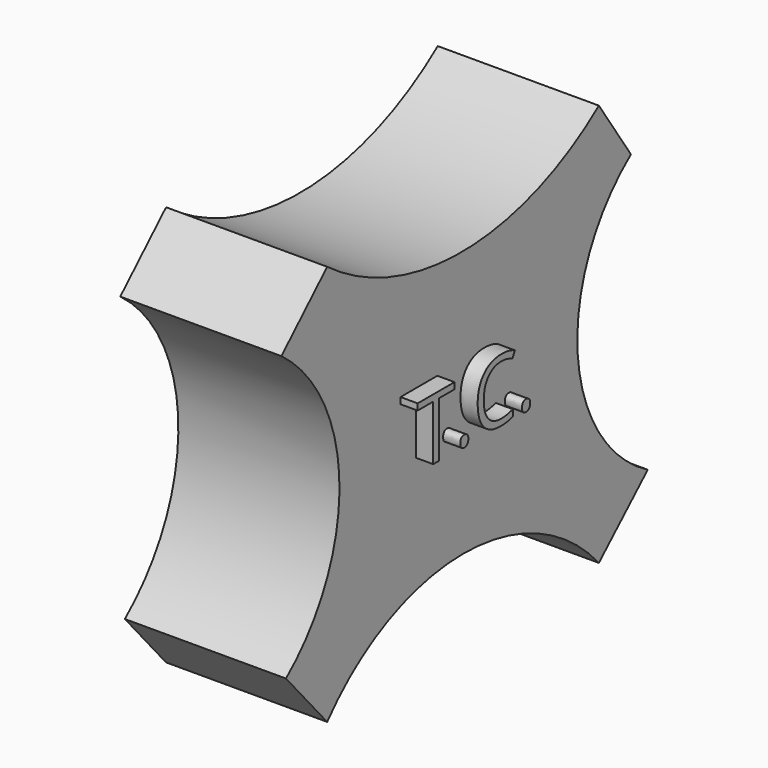
from build123d import *

# Parameters (mm, degrees)
F0_R         = 31.675863552
F0_R_2       = 20.376130664
F1_DEPTH     = 25.4
F0_R_3       = 31.7015587756
F0_R_4       = 20.4227004941
F0_R_5       = 31.6915672548
F0_R_6       = 20.4404132929
F0_R_7       = 31.6458572946
F0_R_8       = 20.0719257162
F3_DEPTH     = 25.4
F4_T         = -2.5
F4_2_T       = -2.5
F4_3_T       = -2.5
F4_4_T       = -2.5
F9_TEXT_SIZE = 13.5690788738
F10_DEPTH    = 28.1


# Not quite as in the source:
# - Text() gives the source's letters only with a copy of the font that has no kerning and outlines rounded to 1/6400 em; it was checked with that copy


with BuildPart() as f1:
    # F0 (on Front) → F1 (new body)
    with BuildSketch(Plane.XZ):
        with Locations((-40.9073680639, 37.5986844301)):
            Circle(F0_R)
        with Locations((-40.9073680639, 37.5986844301)):
            Circle(F0_R_2, mode=Mode.SUBTRACT)
    extrude(amount=F1_DEPTH)

    # F4
    f4_openings = [f1.faces().sort_by_distance(p)[0] for p in [
        (-71.687303, -25.4, 37.598684),
    ]]
    offset(amount=F4_T, openings=f4_openings)


with BuildPart() as f1b:
    # F0 (on Front) → F1, piece 2 (new body)
    with BuildSketch(Plane.XZ):
        with Locations((37.8994755447, 37.5986844301)):
            Circle(F0_R_3)
        with Locations((37.8994755447, 37.5986844301)):
            Circle(F0_R_4, mode=Mode.SUBTRACT)
    extrude(amount=F1_DEPTH)

    # F4#2
    f4_2_openings = [f1b.faces().sort_by_distance(p)[0] for p in [
        (7.094572, -25.4, 37.598684),
    ]]
    offset(amount=F4_2_T, openings=f4_2_openings)


with BuildPart() as f1c:
    # F0 (on Front) → F1, piece 3 (new body)
    with BuildSketch(Plane.XZ):
        with Locations((37.8994755447, -36.696318537)):
            Circle(F0_R_5)
        with Locations((37.8994755447, -36.696318537)):
            Circle(F0_R_6, mode=Mode.SUBTRACT)
    extrude(amount=F1_DEPTH)

    # F4#4
    f4_4_openings = [f1c.faces().sort_by_distance(p)[0] for p in [
        (7.104281, -25.4, -36.696319),
    ]]
    offset(amount=F4_4_T, openings=f4_4_openings)


with BuildPart() as f1d:
    # F0 (on Front) → F1, piece 4 (new body)
    with BuildSketch(Plane.XZ):
        with Locations((-40.9073680639, -36.696318537)):
            Circle(F0_R_7)
        with Locations((-40.9073680639, -36.696318537)):
            Circle(F0_R_8, mode=Mode.SUBTRACT)
    extrude(amount=F1_DEPTH)

    # F4#3
    f4_3_openings = [f1d.faces().sort_by_distance(p)[0] for p in [
        (-71.658145, -25.4, -36.696319),
    ]]
    offset(amount=F4_3_T, openings=f4_3_openings)


with BuildPart() as f3:
    # F2 (on Right) → F3 (new body)
    with BuildSketch(Plane.YZ):
        with BuildLine():
            ThreePointArc((64.6697282791, 31.2821045518), (38.0009545406, 21.9491823139), (11.1292116344, 30.6805260479))
            Line((11.1292116344, 30.6805260479), (2.1055291872, 21.9491823139))
            ThreePointArc((2.1055291872, 21.9491823139), (13.545850262, -0.3859795657), (3.0078974087, -23.1607891619))
            Line((3.0078974087, -23.1607891619), (11.1292116344, -32.4852652848))
            ThreePointArc((11.1292116344, -32.4852652848), (37.8303737781, -20.0358192392), (64.6697282791, -32.1844741702))
            Line((64.6697282791, -32.1844741702), (74.2950066924, -23.1607891619))
            ThreePointArc((74.2950066924, -23.1607891619), (60.495703437, -1.4966005988), (70.9863230586, 21.9491823139))
            Line((70.9863230586, 21.9491823139), (64.6697282791, 31.2821045518))
        make_face()
    extrude(amount=F3_DEPTH)

    # F9 (on Right) → F10 (join)
    with BuildSketch(Plane.YZ):
        with Locations((25.4605337977, -2.9605268501)):
            Text('T.C.', F9_TEXT_SIZE, font='Open Sans', text_align=(TextAlign.LEFT, TextAlign.BOTTOM))
    extrude(amount=F10_DEPTH)


solid = f3.part
